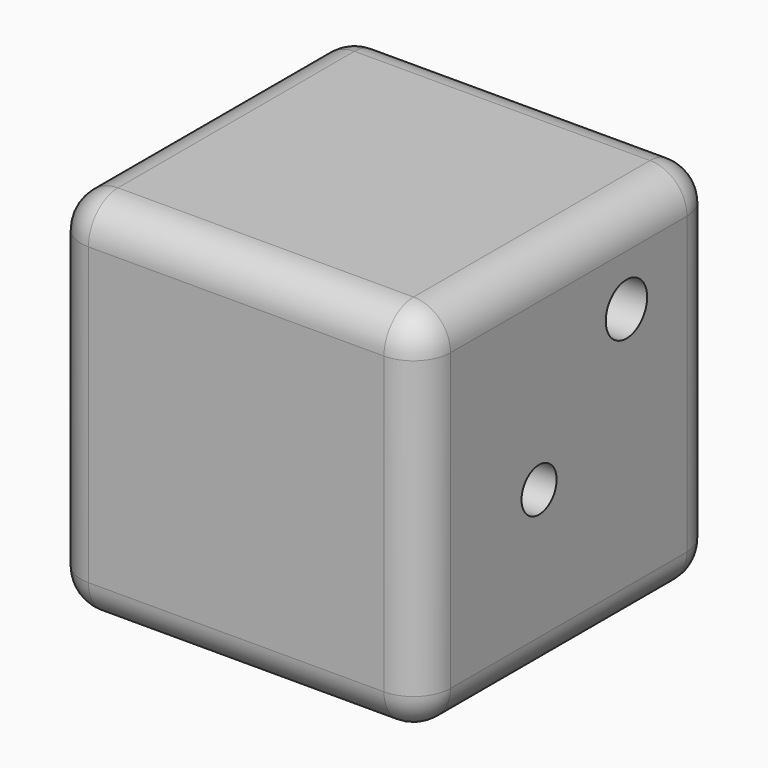
from build123d import *

# Parameters (mm, degrees)
F0_W     = 100
F0_H     = 100
F1_DEPTH = 100
F2_R     = 10
F3_R     = 7.3330548606
F4_DEPTH = 5
F5_R     = 7.0099311872
F5_R_2   = 5.9405048223
F6_DEPTH = 18


# Not quite as in the source:
# - a fillet or chamfer that OpenCascade refuses, or shapes differently, is made with other operations: its cross-section is extruded or revolved along the edge and cut away or added


with BuildPart() as f1:
    # F0 (on Top) → F1 (new body)
    with BuildSketch(Plane.XY):
        Rectangle(F0_W, F0_H)
    extrude(amount=F1_DEPTH)

    # F2
    f2_edges = [f1.edges().sort_by_distance(p)[0] for p in [
        (-50, -50, 50),
        (0, -50, 0),
        (50, -50, 50),
        (-50, 0, 100),
        (0, 50, 100),
        (50, 0, 100),
        (0, -50, 100),
        (-50, 0, 0),
        (-50, 50, 50),
        (0, 50, 0),
        (50, 50, 50),
        (50, 0, 0),
    ]]
    fillet(f2_edges, radius=F2_R)

    # F3 (on face) → F4 (cut)
    with BuildSketch(Plane(origin=(-50, 0, 0), x_dir=(0, -1, 0), z_dir=(-1, 0, 0))):
        with Locations((1.8755461788, 50)):
            Circle(F3_R)
    extrude(amount=-F4_DEPTH, mode=Mode.SUBTRACT)

    # F5 (on face) → F6 (cut)
    with BuildSketch(Plane.YZ.offset(50)):
        with Locations((19.523344934, 76.1831775308)):
            Circle(F5_R)
        with Locations((-10.0353639573, 45.1647788286)):
            Circle(F5_R_2)
    extrude(amount=-F6_DEPTH, mode=Mode.SUBTRACT)

    # F7: fillet of radius 7.2426406871 on 5 edges, made by hand

    # F7_s1 → F7_t2 (revolve)
    with BuildSketch(Plane.XY.offset(50)):
        with BuildLine():
            ThreePointArc((-50, -9.2086010394), (-46.3818180141, -6.5771030138), (-45, -2.3219177396))
            Line((-45, -2.3219177396), (-45, -9.2086010394))
            Line((-45, -9.2086010394), (-50, -9.2086010394))
        make_face()
    revolve(axis=Axis((-45, -1.8755461788, 50), (-1, 0, 0)))


solid = f1.part
